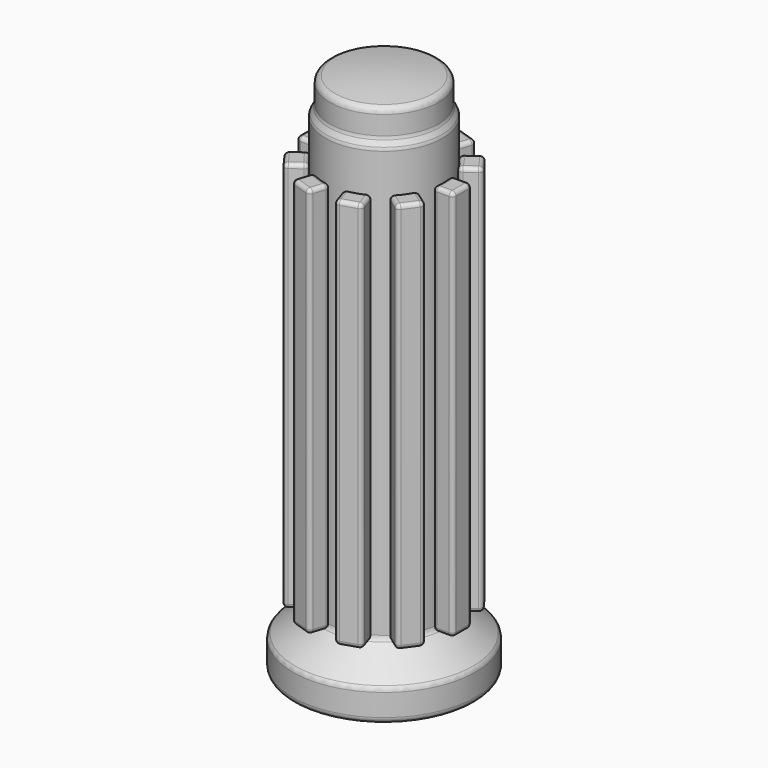
from build123d import *

# Parameters (mm, degrees)
F2_R          = 1.6
F5_END_RADIUS = 15
F4_W          = 6
F4_H          = 100
F5_REACH      = 143.5231135391
F6_R          = 1
F7_COUNT      = 10


with BuildPart() as f1:
    # F0 (on Front) → F1 (revolve)
    with BuildSketch(Plane.XZ):
        with BuildLine():
            ThreePointArc((13.8452994616, 133.5755787269), (6.9591898441, 134.6429573327), (0, 135))
            Line((0, 135), (0, 125))
            Line((0, 125), (10.75, 125))
            Line((10.75, 125), (10.75, 0))
            Line((10.75, 0), (23.3422751482, 0))
            Line((23.3422751482, 0), (23.3422751482, 8))
            Line((23.3422751482, 8), (15, 15))
            Line((15, 15), (15, 125))
            Line((15, 125), (13.8452994616, 127))
            Line((13.8452994616, 127), (13.8452994616, 133.5755787269))
        make_face()
    revolve(axis=Axis((0, 0, 33.5), (0, 0, 1)))

    # F2
    f2_edges = [f1.edges().sort_by_distance(p)[0] for p in [
        (-13.845299, 0, 133.575579),
        (-13.845299, 0, 127),
        (-15, 0, 125),
        (-15, 0, 15),
        (-23.342275, 0, 8),
        (-23.342275, 0, 0),
    ]]
    fillet(f2_edges, radius=F2_R)


with BuildPart() as f5:
    f5_end = (Plane.XY.offset(70.1586867727) * Cylinder(F5_END_RADIUS, 587.6050042205, mode=Mode.PRIVATE)).faces().sort_by_distance((-15, 0, 70.1586867727))[0]
    # F4 (on offset) → F5 (new body, up to the whole of a round face its end follows)
    with BuildSketch(Plane.YZ.offset(20)):
        with Locations((0, 65)):
            Rectangle(F4_W, F4_H)
    f5_long = extrude(amount=-F5_REACH, mode=Mode.PRIVATE)
    add(split(f5_long, bisect_by=f5_end, keep=Keep.ALL, mode=Mode.PRIVATE).solids().sort_by_distance((20, 0, 65))[0])

    # F6
    f6_edges = [f5.edges().sort_by_distance(p)[0] for p in [
        (17.348469, 3, 115),
        (17.348469, -3, 115),
        (20, -3, 65),
        (20, 3, 65),
        (14.696938, 3, 65),
        (14.696938, -3, 65),
        (17.348469, 3, 15),
        (20, 0, 15),
        (14.924042, 1.507634, 15),
        (14.924042, -1.507634, 15),
        (17.348469, -3, 15),
        (14.924042, -1.507634, 115),
        (14.924042, 1.507634, 115),
        (20, 0, 115),
    ]]
    fillet(f6_edges, radius=F6_R)


with BuildPart() as f7_1:
    # F7: instance of F5
    add(f5.part.rotate(Axis((0, 0, 33.5), (0, 0, 1)), 1 * 360 / F7_COUNT))


with BuildPart() as f7_2:
    # F7: instance of F5
    add(f5.part.rotate(Axis((0, 0, 33.5), (0, 0, 1)), 2 * 360 / F7_COUNT))


with BuildPart() as f7_3:
    # F7: instance of F5
    add(f5.part.rotate(Axis((0, 0, 33.5), (0, 0, 1)), 3 * 360 / F7_COUNT))


with BuildPart() as f7_4:
    # F7: instance of F5
    add(f5.part.rotate(Axis((0, 0, 33.5), (0, 0, 1)), 4 * 360 / F7_COUNT))


with BuildPart() as f7_5:
    # F7: instance of F5
    add(f5.part.rotate(Axis((0, 0, 33.5), (0, 0, 1)), 5 * 360 / F7_COUNT))


with BuildPart() as f7_6:
    # F7: instance of F5
    add(f5.part.rotate(Axis((0, 0, 33.5), (0, 0, 1)), 6 * 360 / F7_COUNT))


with BuildPart() as f7_7:
    # F7: instance of F5
    add(f5.part.rotate(Axis((0, 0, 33.5), (0, 0, 1)), 7 * 360 / F7_COUNT))


with BuildPart() as f7_8:
    # F7: instance of F5
    add(f5.part.rotate(Axis((0, 0, 33.5), (0, 0, 1)), 8 * 360 / F7_COUNT))


with BuildPart() as f7_9:
    # F7: instance of F5
    add(f5.part.rotate(Axis((0, 0, 33.5), (0, 0, 1)), 9 * 360 / F7_COUNT))


solid = Compound([f1.part, f5.part, f7_1.part, f7_2.part, f7_3.part, f7_4.part, f7_5.part, f7_6.part, f7_7.part, f7_8.part, f7_9.part])
